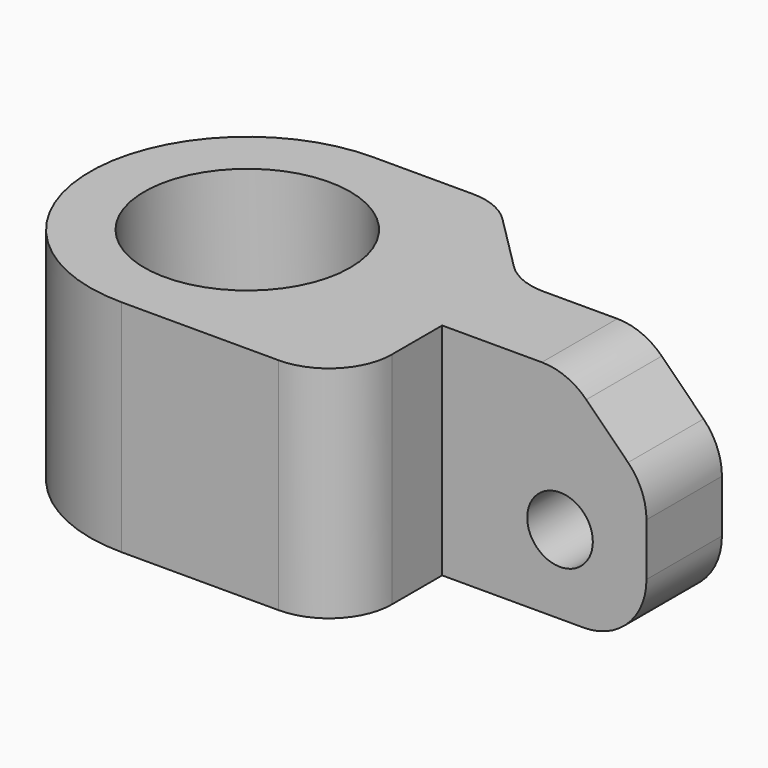
from build123d import *

# Parameters (mm, degrees)
F1_DEPTH  = 17.78
F2_W      = 7.62
F2_H      = 17.78
F3_DEPTH  = 16.51
F4_SIZE   = 6.35
F5_R      = 2.65
F6_DEPTH  = 25.4
F7_R      = 5.08
F12_DEPTH = 17.78
F13_R     = 8.3185
F14_DEPTH = 17.781


# Not quite as in the source:
# - two fillets or chamfers of one size are made in one step
# - a feature names something its author has since deleted; it is built from what else it names


with BuildPart() as f1:
    # F0 (on Top) → F1 (new body)
    with BuildSketch(Plane.XY):
        Polygon((0, 12.7), (0, -12.7), (17.78, -12.7), (17.78, 5.08), (10.16, 12.7), align=None)
    extrude(amount=F1_DEPTH)

    # F2 (on face) → F3 (join)
    with BuildSketch(Plane.YZ.offset(17.78)):
        with Locations((1.27, 8.89)):
            Rectangle(F2_W, F2_H)
    extrude(amount=F3_DEPTH)

    # F4
    f4_edges = [f1.edges().sort_by_distance(p)[0] for p in [
        (34.29, 1.27, 17.78),
    ]]
    chamfer(f4_edges, length=F4_SIZE)

    # F5 (on face) → F6 (cut)
    with BuildSketch(Plane.XZ.offset(2.54)):
        with Locations((27.305, 6.35)):
            Circle(F5_R)
    extrude(amount=-F6_DEPTH, mode=Mode.SUBTRACT)

    # F7
    f7_edges = [f1.edges().sort_by_distance(p)[0] for p in [
        (27.94, 1.27, 17.78),
        (34.29, 1.27, 11.43),
        (17.78, -12.7, 8.89),
        (17.78, 5.08, 8.89),
        (10.16, 12.7, 8.89),
        (34.29, 1.27, 0),
    ]]
    fillet(f7_edges, radius=F7_R)

    # F11 (on face) → F12 (join, through all)
    with BuildSketch(Plane.XY.offset(17.78)):
        with BuildLine():
            Line((0, -12.7), (0, 12.7))
            ThreePointArc((0, 12.7), (-12.7, 0), (0, -12.7))
        make_face()
    extrude(amount=-F12_DEPTH)

    # F13 (on face) → F14 (cut, through all)
    with BuildSketch(Plane.XY.offset(17.78)):
        Circle(F13_R)
    extrude(amount=-F14_DEPTH, mode=Mode.SUBTRACT)


solid = f1.part
